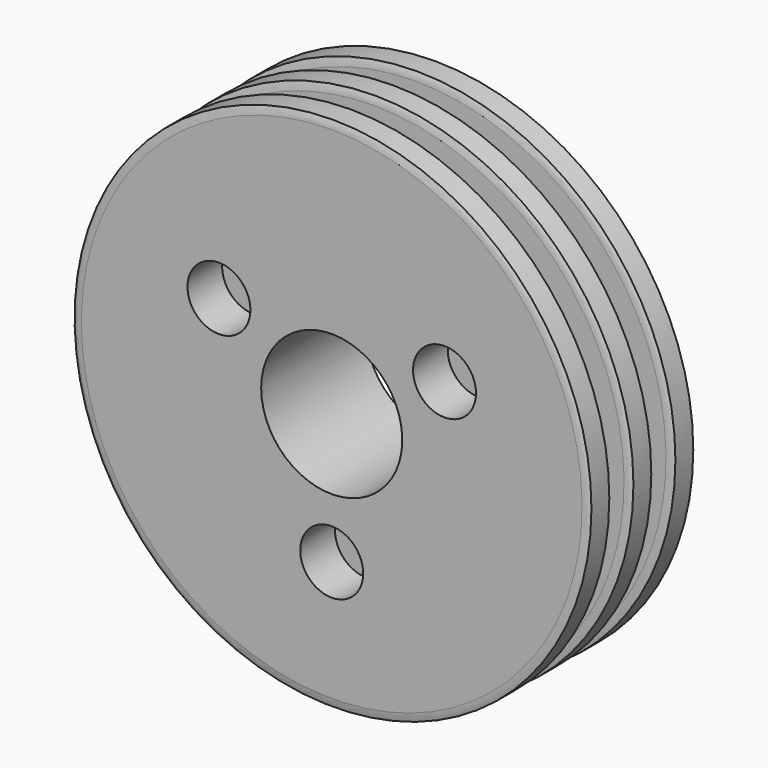
from build123d import *

# Parameters (mm, degrees)
F0_R            = 238.1
F1_DEPTH        = 60.15
F1_DEPTH_BACK   = 60.15
F3_D            = 130
F5_D            = 25
F5_CBORE_D      = 58
F5_CBORE_DEPTH  = 40
F5_COPIES_COUNT = 3
F6_R            = 29
F7_DEPTH        = 40
F7_COPIES_COUNT = 3


# Not quite as in the source:
# - a pattern or mirror of a feature is missing from the dataset's text; its kind, count and spacing are read off the source's solid
# - a feature names something its author has since deleted; it is built from what else it names


with BuildPart() as f1:
    # F0 (on Front) → F1 (new body, two sides)
    with BuildSketch(Plane.XZ) as f1_sk:
        Circle(F0_R)
    extrude(amount=F1_DEPTH)
    extrude(f1_sk.sketch, amount=-F1_DEPTH_BACK)

    # F3 (through all)
    with Locations(Plane.XZ.offset(60.15)):
        with Locations((0, 0)):
            Hole(F3_D / 2)

    # F5 (through all)
    with Locations(Plane.XZ.offset(60.15)):
        with Locations((0, -120)):
            f5 = CounterBoreHole(F5_D / 2, F5_CBORE_D / 2, F5_CBORE_DEPTH)

    # F5_copies: F5 ×3 about axis
    f5_copies_axis = Axis((0, 0, 0), (0, 1, 0))
    for i in range(1, F5_COPIES_COUNT):
        add(f5.rotate(f5_copies_axis, i * 360 / F5_COPIES_COUNT), mode=Mode.SUBTRACT)

    # F6 (on face) → F7 (cut)
    with BuildSketch(Plane(origin=(0, 60.15, 0), x_dir=(-1, 0, 0), z_dir=(0, 1, 0))):
        with Locations((0, 120)):
            Circle(F6_R)
    f7 = extrude(amount=-F7_DEPTH, mode=Mode.SUBTRACT)

    # F7_copies: F7 ×3 about axis
    f7_copies_axis = Axis((0, 0, 0), (0, 1, 0))
    for i in range(1, F7_COPIES_COUNT):
        add(f7.rotate(f7_copies_axis, i * 360 / F7_COPIES_COUNT), mode=Mode.SUBTRACT)

    # F8 (on Right) → F9 (revolve, cut)
    with BuildSketch(Plane.YZ):
        with BuildLine():
            Line((-36.55, 205.69), (-11.8, 205.69))
            Line((-11.8, 205.69), (-11.8, 230.69))
            ThreePointArc((-11.8, 230.69), (-11.4200720085, 234.4705976243), (-10.295482274, 238.1))
            Line((-10.295482274, 238.1), (10.295482274, 238.1))
            ThreePointArc((10.295482274, 238.1), (11.4200720085, 234.4705976243), (11.8, 230.69))
            Line((11.8, 230.69), (11.8, 205.69))
            Line((11.8, 205.69), (36.55, 205.69))
            Line((36.55, 205.69), (36.55, 230.69))
            ThreePointArc((36.55, 230.69), (36.9299279915, 234.4705976243), (38.054517726, 238.1))
            Line((38.054517726, 238.1), (58.645482274, 238.1))
            ThreePointArc((58.645482274, 238.1), (59.7700720085, 234.4705976243), (60.15, 230.69))
            Line((60.15, 230.69), (60.15, 223.28))
            Line((60.15, 223.28), (86.0586377919, 223.28))
            Line((86.0586377919, 223.28), (86.0586377919, 283.6410403252))
            Line((86.0586377919, 283.6410403252), (-71.6444390953, 283.6410403252))
            Line((-71.6444390953, 283.6410403252), (-71.6444390953, 224.8791903257))
            Line((-71.6444390953, 224.8791903257), (-60.15, 224.8791903257))
            Line((-60.15, 224.8791903257), (-60.15, 230.69))
            ThreePointArc((-60.15, 230.69), (-59.7700720085, 234.4705976243), (-58.645482274, 238.1))
            Line((-58.645482274, 238.1), (-38.054517726, 238.1))
            ThreePointArc((-38.054517726, 238.1), (-36.9299279915, 234.4705976243), (-36.55, 230.69))
            Line((-36.55, 230.69), (-36.55, 205.69))
        make_face()
    revolve(axis=Axis((0, 0, 0), (0, 1, 0)), mode=Mode.SUBTRACT)


solid = f1.part
